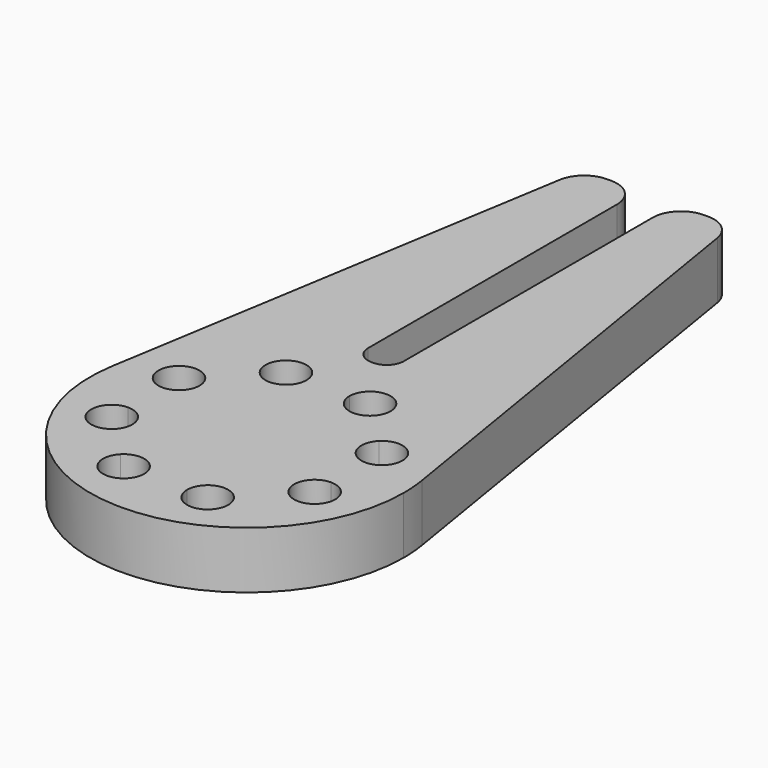
from build123d import *

# Parameters (mm, degrees)
F1_DEPTH = 5.08
F3_DEPTH = 25.4
F4_R     = 2.54
F5_R     = 1.524


with BuildPart() as f1:
    # F0 (on Top) → F1 (new body)
    with BuildSketch(Plane.XY):
        with BuildLine():
            ThreePointArc((-13.7862916745, 2.2581102419), (-1.1327853518, -13.9239971756), (13.97, 0))
            ThreePointArc((13.97, 0), (13.9239971756, 1.1327853518), (13.7862916745, 2.2581102419))
            ThreePointArc((13.7862916745, 2.2581102419), (9.0447526202, 10.646753028), (0, 13.97))
            ThreePointArc((0, 13.97), (-9.0447526202, 10.646753028), (-13.7862916745, 2.2581102419))
        make_face()
        with BuildLine():
            Line((-6.6675, 45.72), (-13.7862916745, 2.2581102419))
            ThreePointArc((-13.7862916745, 2.2581102419), (-9.0447526202, 10.646753028), (0, 13.97))
            Line((0, 13.97), (-1.5875, 13.97))
            Line((-1.5875, 13.97), (-1.5875, 45.72))
            Line((-1.5875, 45.72), (-6.6675, 45.72))
        make_face()
        with BuildLine():
            ThreePointArc((0, 13.97), (9.0447526202, 10.646753028), (13.7862916745, 2.2581102419))
            Line((13.7862916745, 2.2581102419), (6.6675, 45.72))
            Line((6.6675, 45.72), (1.5875, 45.72))
            Line((1.5875, 45.72), (1.5875, 13.97))
            Line((1.5875, 13.97), (0, 13.97))
        make_face()
    extrude(amount=F1_DEPTH)

    # F2 (on face) → F3 (cut)
    with BuildSketch(Plane.XY.offset(5.08)):
        with BuildLine():
            Line((-3.7422612851, 9.0346179484), (-1.9134612851, 9.0346179484))
            ThreePointArc((-1.9134612851, 9.0346179484), (-4.4421127462, 10.7242088375), (-5.0354181665, 7.741461067))
            Line((-5.0354181665, 7.741461067), (-3.7422612851, 9.0346179484))
        make_face()
        with BuildLine():
            ThreePointArc((-5.0354181665, 7.741461067), (-3.042409824, 7.3450270594), (-1.9134612851, 9.0346179484))
            Line((-1.9134612851, 9.0346179484), (-3.7422612851, 9.0346179484))
            Line((-3.7422612851, 9.0346179484), (-5.0354181665, 7.741461067))
        make_face()
        with BuildLine():
            Line((3.7422612851, 9.0346179484), (5.0354181665, 7.741461067))
            ThreePointArc((5.0354181665, 7.741461067), (5.4318521742, 8.3347664873), (5.5710612851, 9.0346179484))
            ThreePointArc((5.5710612851, 9.0346179484), (3.7422612851, 10.8634179484), (1.9134612851, 9.0346179484))
            Line((1.9134612851, 9.0346179484), (3.7422612851, 9.0346179484))
        make_face()
        with BuildLine():
            ThreePointArc((1.9134612851, 9.0346179484), (3.042409824, 7.3450270594), (5.0354181665, 7.741461067))
            Line((5.0354181665, 7.741461067), (3.7422612851, 9.0346179484))
            Line((3.7422612851, 9.0346179484), (1.9134612851, 9.0346179484))
        make_face()
        with BuildLine():
            Line((7.741461067, 5.0354181665), (9.0346179484, 3.7422612851))
            Line((9.0346179484, 3.7422612851), (9.0346179484, 1.9134612851))
            ThreePointArc((9.0346179484, 1.9134612851), (10.3277748299, 2.4491044037), (10.8634179484, 3.7422612851))
            ThreePointArc((10.8634179484, 3.7422612851), (9.7344694095, 5.4318521742), (7.741461067, 5.0354181665))
        make_face()
        with BuildLine():
            Line((9.0346179484, 1.9134612851), (9.0346179484, 3.7422612851))
            Line((9.0346179484, 3.7422612851), (7.741461067, 5.0354181665))
            ThreePointArc((7.741461067, 5.0354181665), (7.3450270594, 3.042409824), (9.0346179484, 1.9134612851))
        make_face()
        with BuildLine():
            ThreePointArc((10.8634179484, -3.7422612851), (10.3277748299, -2.4491044037), (9.0346179484, -1.9134612851))
            Line((9.0346179484, -1.9134612851), (9.0346179484, -3.7422612851))
            Line((9.0346179484, -3.7422612851), (7.741461067, -5.0354181665))
            ThreePointArc((7.741461067, -5.0354181665), (9.7344694095, -5.4318521742), (10.8634179484, -3.7422612851))
        make_face()
        with BuildLine():
            Line((9.0346179484, -3.7422612851), (9.0346179484, -1.9134612851))
            ThreePointArc((9.0346179484, -1.9134612851), (7.3450270594, -3.042409824), (7.741461067, -5.0354181665))
            Line((7.741461067, -5.0354181665), (9.0346179484, -3.7422612851))
        make_face()
        with BuildLine():
            ThreePointArc((5.5710612851, -9.0346179484), (5.4318521742, -8.3347664873), (5.0354181665, -7.741461067))
            Line((5.0354181665, -7.741461067), (3.7422612851, -9.0346179484))
            Line((3.7422612851, -9.0346179484), (1.9134612851, -9.0346179484))
            ThreePointArc((1.9134612851, -9.0346179484), (3.7422612851, -10.8634179484), (5.5710612851, -9.0346179484))
        make_face()
        with BuildLine():
            Line((3.7422612851, -9.0346179484), (5.0354181665, -7.741461067))
            ThreePointArc((5.0354181665, -7.741461067), (3.042409824, -7.3450270594), (1.9134612851, -9.0346179484))
            Line((1.9134612851, -9.0346179484), (3.7422612851, -9.0346179484))
        make_face()
        with BuildLine():
            ThreePointArc((-5.0354181665, -7.741461067), (-4.4421127462, -10.7242088375), (-1.9134612851, -9.0346179484))
            Line((-1.9134612851, -9.0346179484), (-3.7422612851, -9.0346179484))
            Line((-3.7422612851, -9.0346179484), (-5.0354181665, -7.741461067))
        make_face()
        with BuildLine():
            Line((-3.7422612851, -9.0346179484), (-1.9134612851, -9.0346179484))
            ThreePointArc((-1.9134612851, -9.0346179484), (-3.042409824, -7.3450270594), (-5.0354181665, -7.741461067))
            Line((-5.0354181665, -7.741461067), (-3.7422612851, -9.0346179484))
        make_face()
        with BuildLine():
            Line((-9.0346179484, -3.7422612851), (-7.741461067, -5.0354181665))
            ThreePointArc((-7.741461067, -5.0354181665), (-7.3450270594, -4.4421127462), (-7.2058179484, -3.7422612851))
            ThreePointArc((-7.2058179484, -3.7422612851), (-7.741461067, -2.4491044037), (-9.0346179484, -1.9134612851))
            Line((-9.0346179484, -1.9134612851), (-9.0346179484, -3.7422612851))
        make_face()
        with BuildLine():
            ThreePointArc((-9.0346179484, -1.9134612851), (-10.7242088375, -4.4421127462), (-7.741461067, -5.0354181665))
            Line((-7.741461067, -5.0354181665), (-9.0346179484, -3.7422612851))
            Line((-9.0346179484, -3.7422612851), (-9.0346179484, -1.9134612851))
        make_face()
        with BuildLine():
            Line((-9.0346179484, 3.7422612851), (-7.741461067, 5.0354181665))
            ThreePointArc((-7.741461067, 5.0354181665), (-10.7242088375, 4.4421127462), (-9.0346179484, 1.9134612851))
            Line((-9.0346179484, 1.9134612851), (-9.0346179484, 3.7422612851))
        make_face()
        with BuildLine():
            ThreePointArc((-7.2058179484, 3.7422612851), (-7.3450270594, 4.4421127462), (-7.741461067, 5.0354181665))
            Line((-7.741461067, 5.0354181665), (-9.0346179484, 3.7422612851))
            Line((-9.0346179484, 3.7422612851), (-9.0346179484, 1.9134612851))
            ThreePointArc((-9.0346179484, 1.9134612851), (-7.741461067, 2.4491044037), (-7.2058179484, 3.7422612851))
        make_face()
    extrude(amount=-F3_DEPTH, mode=Mode.SUBTRACT)

    # F4
    f4_edges = [f1.edges().sort_by_distance(p)[0] for p in [
        (1.5875, 45.72, 2.54),
        (-1.5875, 45.72, 2.54),
        (-6.6675, 45.72, 2.54),
        (6.6675, 45.72, 2.54),
    ]]
    fillet(f4_edges, radius=F4_R)

    # F5
    f5_edges = [f1.edges().sort_by_distance(p)[0] for p in [
        (-1.5875, 13.97, 2.54),
        (1.5875, 13.97, 2.54),
    ]]
    fillet(f5_edges, radius=F5_R)


solid = f1.part
